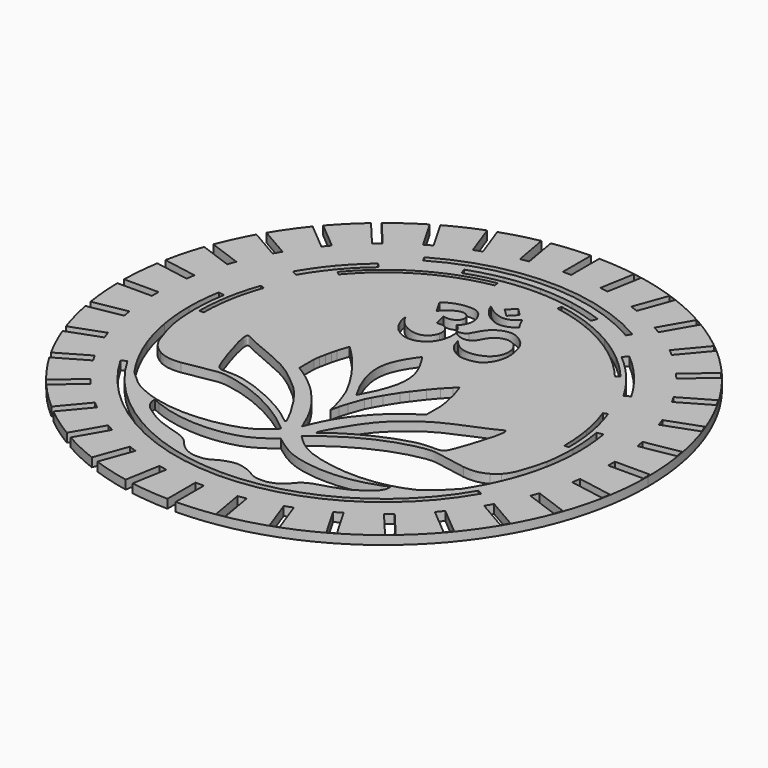
from build123d import *

# Parameters (mm, degrees)
F0_W     = 20
F0_H     = 4.75
F1_DEPTH = 5
F4_DEPTH = 12.5
F5_DEPTH = 12.5


with BuildPart() as f1:
    # F0 (on Top) → F1 (new body)
    with BuildSketch(Plane.XY):
        with BuildLine():
            ThreePointArc((1.597222, -149.991496), (106.629225, -105.499803), (150, 0))
            ThreePointArc((150, 0), (106.902409, 105.222978), (2.375, 149.981197))
            Line((2.375, 149.981197), (2.375, 130))
            Line((2.375, 130), (0, 130))
            Line((0, 130), (-2.375, 130))
            Line((-2.375, 130), (-2.375, 149.981197))
            ThreePointArc((-2.375, 149.981197), (-13.070418, 149.429462), (-23.699208, 148.115993))
            Line((-23.699208, 148.115993), (-20.241253, 128.504952))
            Line((-20.241253, 128.504952), (-24.91909, 127.680123))
            Line((-24.91909, 127.680123), (-28.377078, 147.291349))
            ThreePointArc((-28.377078, 147.291349), (-38.808675, 144.892673), (-49.042654, 141.756192))
            Line((-49.042654, 141.756192), (-42.254302, 123.105346))
            Line((-42.254302, 123.105346), (-46.717841, 121.480751))
            Line((-46.717841, 121.480751), (-53.506448, 140.132295))
            ThreePointArc((-53.506448, 140.132295), (-63.358495, 135.962131), (-72.88825, 131.100355))
            Line((-72.88825, 131.100355), (-62.995291, 113.965247))
            Line((-62.995291, 113.965247), (-67.108912, 111.590247))
            Line((-67.108912, 111.590247), (-77.002696, 128.726784))
            ThreePointArc((-77.002696, 128.726784), (-85.977844, 122.913833), (-94.516059, 116.476241))
            Line((-94.516059, 116.476241), (-81.834016, 101.362371))
            Line((-81.834016, 101.362371), (-85.472728, 98.30913))
            Line((-85.472728, 98.30913), (-98.156622, 113.425207))
            ThreePointArc((-98.156622, 113.425207), (-105.984694, 106.147278), (-113.274614, 98.330371))
            Line((-113.274614, 98.330371), (-98.198073, 85.679651))
            Line((-98.198073, 85.679651), (-101.251314, 82.04094))
            Line((-101.251314, 82.04094), (-116.331225, 94.694488))
            ThreePointArc((-116.331225, 94.694488), (-122.777115, 86.172966), (-128.600028, 77.2142))
            Line((-128.600028, 77.2142), (-111.590247, 67.393598))
            Line((-111.590247, 67.393598), (-113.965247, 63.279977))
            Line((-113.965247, 63.279977), (-130.980362, 73.103658))
            ThreePointArc((-130.980362, 73.103658), (-135.850845, 63.596761), (-140.032397, 53.767349))
            Line((-140.032397, 53.767349), (-121.603624, 47.059825))
            Line((-121.603624, 47.059825), (-123.22822, 42.596285))
            Line((-123.22822, 42.596285), (-141.664608, 49.306581))
            ThreePointArc((-141.664608, 49.306581), (-144.813896, 39.101606), (-147.229077, 28.698413))
            Line((-147.229077, 28.698413), (-127.933953, 25.296162))
            Line((-127.933953, 25.296162), (-128.758781, 20.618325))
            Line((-128.758781, 20.618325), (-148.063929, 24.022344))
            ThreePointArc((-148.063929, 24.022344), (-149.397831, 13.427143), (-149.974534, 2.763889))
            Line((-149.974534, 2.763889), (-130.388889, 2.763889))
            Line((-130.388889, 2.763889), (-130.388889, -1.986111))
            Line((-130.388889, -1.986111), (-149.986851, -1.986111))
            ThreePointArc((-149.986851, -1.986111), (-149.465453, -12.65221), (-148.186514, -23.254183))
            Line((-148.186514, -23.254183), (-128.893841, -19.852364))
            Line((-128.893841, -19.852364), (-128.069012, -24.530201))
            Line((-128.069012, -24.530201), (-147.375921, -27.93453))
            ThreePointArc((-147.375921, -27.93453), (-145.014723, -38.350099), (-141.918401, -48.571261))
            Line((-141.918401, -48.571261), (-123.494235, -41.865413))
            Line((-123.494235, -41.865413), (-121.86964, -46.328953))
            Line((-121.86964, -46.328953), (-140.309338, -53.040454))
            ThreePointArc((-140.309338, -53.040454), (-136.17882, -62.891405), (-131.357711, -72.423421))
            Line((-131.357711, -72.423421), (-114.354136, -62.606402))
            Line((-114.354136, -62.606402), (-111.979136, -66.720023))
            Line((-111.979136, -66.720023), (-128.99871, -76.546279))
            ThreePointArc((-128.99871, -76.546279), (-123.222343, -85.535105), (-116.820743, -94.089925))
            Line((-116.820743, -94.089925), (-101.75126, -81.445128))
            Line((-101.75126, -81.445128), (-98.698019, -85.083839))
            Line((-98.698019, -85.083839), (-113.783001, -97.741642))
            ThreePointArc((-113.783001, -97.741642), (-106.533732, -105.596231), (-98.743524, -112.914642))
            Line((-98.743524, -112.914642), (-86.06854, -97.809184))
            Line((-86.06854, -97.809184), (-82.429829, -100.862425))
            Line((-82.429829, -100.862425), (-95.118795, -115.984546))
            ThreePointArc((-95.118795, -115.984546), (-86.6141, -122.466313), (-77.669239, -128.325716))
            Line((-77.669239, -128.325716), (-67.782487, -111.201358))
            Line((-67.782487, -111.201358), (-63.668866, -113.576358))
            Line((-63.668866, -113.576358), (-73.56711, -130.720619))
            ThreePointArc((-73.56711, -130.720619), (-64.062721, -135.631736), (-54.23246, -139.852924))
            Line((-54.23246, -139.852924), (-47.448714, -121.214735))
            Line((-47.448714, -121.214735), (-42.985174, -122.839331))
            Line((-42.985174, -122.839331), (-49.777091, -141.499969))
            ThreePointArc((-49.777091, -141.499969), (-39.559543, -144.689469), (-29.140556, -147.142203))
            Line((-29.140556, -147.142203), (-25.685051, -127.545064))
            Line((-25.685051, -127.545064), (-21.007214, -128.369892))
            Line((-21.007214, -128.369892), (-24.466964, -147.991107))
            ThreePointArc((-24.466964, -147.991107), (-13.845159, -149.359672), (-3.152778, -149.966863))
            Line((-3.152778, -149.966863), (-3.152778, -130))
            Line((-3.152778, -130), (1.597222, -130))
            Line((1.597222, -130), (1.597222, -149.991496))
        make_face()
        Polygon((24.141312, -127.680123), (27.614275, -147.376278), (22.936439, -148.201107), (19.463475, -128.504952), align=None, mode=Mode.SUBTRACT)
        Polygon((45.940064, -121.480751), (52.780467, -140.274603), (48.316927, -141.899199), (41.476524, -123.105346), align=None, mode=Mode.SUBTRACT)
        Polygon((66.331134, -111.590247), (76.331134, -128.910755), (72.217513, -131.285755), (62.217513, -113.965247), align=None, mode=Mode.SUBTRACT)
        Polygon((84.69495, -98.30913), (97.550702, -113.630019), (93.911991, -116.68326), (81.056239, -101.362371), align=None, mode=Mode.SUBTRACT)
        Polygon((100.473536, -82.04094), (115.794425, -94.896692), (112.741184, -98.535403), (97.420295, -85.679651), align=None, mode=Mode.SUBTRACT)
        Polygon((113.187469, -63.279977), (130.507977, -73.279977), (128.132977, -77.393598), (110.812469, -67.393598), align=None, mode=Mode.SUBTRACT)
        Polygon((122.450442, -42.596285), (141.244294, -49.436688), (139.619699, -53.900227), (120.825846, -47.059825), align=None, mode=Mode.SUBTRACT)
        Polygon((127.981004, -20.618325), (147.677159, -24.091289), (146.85233, -28.769126), (127.156175, -25.296162), align=None, mode=Mode.SUBTRACT)
        with Locations((139.611111, -0.388889)):
            Rectangle(F0_W, F0_H, mode=Mode.SUBTRACT)
        Polygon((127.291234, 24.530201), (146.987389, 28.003164), (147.812218, 23.325327), (128.116063, 19.852364), align=None, mode=Mode.SUBTRACT)
        Polygon((121.091862, 46.328953), (139.885714, 53.169355), (141.51031, 48.705816), (122.716457, 41.865413), align=None, mode=Mode.SUBTRACT)
        Polygon((111.201358, 66.720023), (128.521866, 76.720023), (130.896866, 72.606402), (113.576358, 62.606402), align=None, mode=Mode.SUBTRACT)
        Polygon((20.229437, 128.369892), (23.7024, 148.066048), (28.380237, 147.241219), (24.907273, 127.545064), align=None, mode=Mode.SUBTRACT)
        Polygon((62.891088, 113.576358), (72.891088, 130.896866), (77.004709, 128.521866), (67.004709, 111.201358), align=None, mode=Mode.SUBTRACT)
        Polygon((42.207396, 122.839331), (49.047799, 141.633183), (53.511339, 140.008587), (46.670936, 121.214735), align=None, mode=Mode.SUBTRACT)
        Polygon((97.920241, 85.083839), (113.24113, 97.939591), (116.294371, 94.30088), (100.973482, 81.445128), align=None, mode=Mode.SUBTRACT)
        Polygon((81.652051, 100.862425), (94.507803, 116.183314), (98.146514, 113.130073), (85.290762, 97.809184), align=None, mode=Mode.SUBTRACT)
    extrude(amount=F1_DEPTH)

    # F3 (on face) → F4 (cut, symmetric)
    with BuildSketch(Plane(origin=(0, 0, 0), x_dir=(1, 0, 0), z_dir=(0, 0, -1))):
        with BuildLine():
            ThreePointArc((-57.608503, 99.780855), (-29.820356, 111.291082), (0, 115.217007))
            Line((0, 115.217007), (0, 118.357057))
            ThreePointArc((0, 118.357057), (-30.63306, 114.324138), (-59.178528, 102.500218))
            Line((-59.178528, 102.500218), (-57.608503, 99.780855))
        make_face()
        with BuildLine():
            ThreePointArc((0, 115.217007), (29.820356, 111.291082), (57.608503, 99.780855))
            Line((57.608503, 99.780855), (59.178528, 102.500218))
            ThreePointArc((59.178528, 102.500218), (30.63306, 114.324138), (0, 118.357057))
            Line((0, 118.357057), (0, 115.217007))
        make_face()
        with BuildLine():
            ThreePointArc((-99.780855, 57.608503), (-81.470727, 81.470727), (-57.608503, 99.780855))
            Line((-57.608503, 99.780855), (-59.178528, 102.500218))
            ThreePointArc((-59.178528, 102.500218), (-83.691077, 83.691077), (-102.500218, 59.178528))
            Line((-102.500218, 59.178528), (-99.780855, 57.608503))
        make_face()
        with BuildLine():
            ThreePointArc((57.608503, 99.780855), (81.470727, 81.470727), (99.780855, 57.608503))
            Line((99.780855, 57.608503), (102.500218, 59.178528))
            ThreePointArc((102.500218, 59.178528), (83.691077, 83.691077), (59.178528, 102.500218))
            Line((59.178528, 102.500218), (57.608503, 99.780855))
        make_face()
        with BuildLine():
            Line((59.178528, -102.500218), (57.608503, -99.780855))
            ThreePointArc((57.608503, -99.780855), (0, -115.217007), (-57.608503, -99.780855))
            Line((-57.608503, -99.780855), (-59.178528, -102.500218))
            ThreePointArc((-59.178528, -102.500218), (0, -118.357057), (59.178528, -102.500218))
        make_face()
    extrude(amount=F4_DEPTH, both=True, mode=Mode.SUBTRACT)

    # F2 (on Top) → F5 (cut, symmetric)
    with BuildSketch(Plane.XY):
        with BuildLine():
            add(Edge.make_bspline(
                [(-26.703293, 72.772757), (-22.478819, 76.516569), (-13.505565, 78.302662), (-8.586049, 77.175751), (-6.499787, 75.175449)],
                knots=[0, 0, 0, 0, 0.581389, 1, 1, 1, 1], degree=3))
            add(Edge.make_bspline(
                [(-26.703293, 72.772757), (-25.355081, 70.373524), (-24.053074, 68.074924), (-22.704862, 65.675691)],
                knots=[0, 0, 0, 0, 8.145907, 8.145907, 8.145907, 8.145907], degree=3))
            add(Edge.make_bspline(
                [(-8.665677, 69.281735), (-9.783125, 71.251235), (-13.605188, 73.021978), (-19.772128, 68.764412), (-21.8962, 66.595492), (-22.704862, 65.675691)],
                knots=[0, 0, 0, 0, 0.332513, 0.707051, 1, 1, 1, 1], degree=3))
            add(Edge.make_bspline(
                [(-17.057454, 63.531227), (-16.037357, 63.26761), (-13.208657, 62.663421), (-8.578156, 65.063049), (-8.277197, 67.8832), (-8.665677, 69.281735)],
                knots=[0, 0, 0, 0, 0.320478, 0.676624, 1, 1, 1, 1], degree=3))
            add(Edge.make_bspline(
                [(-15.444824, 56.62287), (-15.982367, 58.925656), (-16.519911, 61.228442), (-17.057454, 63.531227)],
                knots=[0, 0, 0, 0, 7.09408, 7.09408, 7.09408, 7.09408], degree=3))
            add(Edge.make_bspline(
                [(-7.991881, 49.536288), (-7.594286, 52.1168), (-9.312323, 56.461701), (-12.466869, 56.971069), (-15.444824, 56.62287)],
                knots=[0, 0, 0, 0, 0.508663, 1, 1, 1, 1], degree=3))
            add(Edge.make_bspline(
                [(-29.753646, 52.613709), (-28.553318, 49.875669), (-25.266547, 45.549492), (-15.312613, 41.506839), (-9.279541, 45.082696), (-7.991881, 49.536288)],
                knots=[0, 0, 0, 0, 0.315633, 0.654187, 1, 1, 1, 1], degree=3))
            add(Edge.make_bspline(
                [(-24.630969, 41.01808), (-26.457644, 42.921507), (-29.062424, 47.330559), (-29.671244, 50.90585), (-29.753646, 52.613709)],
                knots=[0, 0, 0, 0, 0.547939, 1, 1, 1, 1], degree=3))
            add(Edge.make_bspline(
                [(-2.568085, 54.219991), (-2.478607, 52.847017), (-2.376396, 49.888119), (-3.428155, 45.220364), (-6.026805, 41.186891), (-8.67628, 38.939767), (-12.542173, 37.245592), (-16.577244, 36.933956), (-20.991081, 38.095522), (-23.327493, 39.967105), (-24.630969, 41.01808)],
                knots=[0, 0, 0, 0, 0.124945, 0.257135, 0.38776, 0.499819, 0.62179, 0.742926, 0.869214, 1, 1, 1, 1], degree=3))
            add(Edge.make_bspline(
                [(19.814819, 63.531227), (18.768377, 63.637798), (16.005393, 63.028155), (12.611332, 61.256179), (10.143988, 57.191455), (9.248884, 55.056364), (7.358842, 52.780087), (3.834369, 51.865212), (0.587411, 52.562146), (-1.582146, 53.720386), (-2.568085, 54.219991)],
                knots=[0, 0, 0, 0, 0.129745, 0.263756, 0.408093, 0.51199, 0.624075, 0.750013, 0.873115, 1, 1, 1, 1], degree=3))
            add(Edge.make_bspline(
                [(2.779092, 49.023379), (3.524531, 48.139071), (5.061174, 46.316162), (8.41181, 44.063753), (12.929503, 42.815322), (18.32591, 43.76921), (22.435249, 45.5927), (25.43589, 48.537302), (27.143227, 52.461491), (27.136221, 57.967533), (24.075212, 62.45953), (21.486653, 63.253537), (19.814819, 63.531227)],
                knots=[0, 0, 0, 0, 0.088628, 0.182697, 0.284338, 0.39447, 0.494693, 0.589628, 0.686383, 0.795998, 0.901602, 1, 1, 1, 1], degree=3))
            add(Edge.make_bspline(
                [(29.083719, 56.863476), (29.346624, 55.498138), (29.946058, 51.835685), (28.788033, 45.586509), (26.804438, 42.261139), (24.342062, 39.384339), (20.845119, 37.95796), (15.851711, 37.257572), (10.876852, 37.898382), (5.88339, 41.831034), (3.659308, 45.212339), (3.069999, 47.763849), (2.779092, 49.023379)],
                knots=[0, 0, 0, 0, 0.104459, 0.221836, 0.313636, 0.401904, 0.491563, 0.595441, 0.699744, 0.815334, 0.908841, 1, 1, 1, 1], degree=3))
            add(Edge.make_bspline(
                [(2.009738, 57.852648), (3.693849, 60.468544), (5.726443, 66.167234), (15.863503, 71.372649), (23.67625, 67.30442), (27.644872, 62.48758), (28.609513, 58.71806), (29.083719, 56.863476)],
                knots=[0, 0, 0, 0, 0.217271, 0.445619, 0.650372, 0.828044, 1, 1, 1, 1], degree=3))
            add(Edge.make_bspline(
                [(-3.712958, 56.326561), (-3.045915, 55.933479), (-1.286406, 55.653666), (1.058829, 56.729218), (2.009738, 57.852648)],
                knots=[0, 0, 0, 0, 0.436713, 1, 1, 1, 1], degree=3))
            add(Edge.make_bspline(
                [(-7.261419, 60.502313), (-6.41553, 60.155282), (-4.686406, 58.60729), (-4.184914, 57.1977), (-3.712958, 56.326561)],
                knots=[0, 0, 0, 0, 0.519128, 1, 1, 1, 1], degree=3))
            add(Edge.make_bspline(
                [(-6.499787, 75.175449), (-4.902218, 72.844208), (-2.580657, 68.502349), (-4.714982, 62.642939), (-7.261419, 60.502313)],
                knots=[0, 0, 0, 0, 0.481783, 1, 1, 1, 1], degree=3))
        make_face()
        with BuildLine():
            add(Edge.make_bspline(
                [(-6.618558, 84.143944), (-3.438113, 81.399173), (3.917643, 77.195458), (9.457943, 79.525754), (12.442335, 82.793348)],
                knots=[0, 0, 0, 0, 0.52571, 1, 1, 1, 1], degree=3))
            add(Edge.make_bspline(
                [(15.862403, 76.34531), (13.959511, 74.267434), (7.616297, 70.926623), (-2.460375, 76.240025), (-5.876792, 82.00591), (-6.618558, 84.143944)],
                knots=[0, 0, 0, 0, 0.325363, 0.68111, 1, 1, 1, 1], degree=3))
            add(Edge.make_bspline(
                [(12.442335, 82.793348), (13.444393, 80.418892), (14.272179, 78.545474), (15.862403, 76.34531)],
                knots=[0, 0, 0, 0, 7.298908, 7.298908, 7.298908, 7.298908], degree=3))
        make_face()
        Polygon((8.61929, 85.590638), (4.404083, 89.894883), (0.156227, 85.538112), (4.46861, 81.333535), align=None)
        with BuildLine():
            Line((18.667179, 105.866833), (19.274948, 109.313661))
            ThreePointArc((19.274948, 109.313661), (9.674287, 110.577611), (0, 111))
            Line((0, 111), (0, 107.5))
            ThreePointArc((0, 107.5), (9.369242, 107.09093), (18.667179, 105.866833))
        make_face()
        with BuildLine():
            Line((0, 107.5), (0, 111))
            ThreePointArc((0, 111), (-9.674287, 110.577611), (-19.274948, 109.313661))
            Line((-19.274948, 109.313661), (-18.667179, 105.866833))
            ThreePointArc((-18.667179, 105.866833), (-9.369242, 107.09093), (0, 107.5))
        make_face()
        with BuildLine():
            Line((-18.667179, 105.866833), (-19.274948, 109.313661))
            ThreePointArc((-19.274948, 109.313661), (-28.728914, 107.217767), (-37.964236, 104.305881))
            Line((-37.964236, 104.305881), (-36.767165, 101.016957))
            ThreePointArc((-36.767165, 101.016957), (-27.823047, 103.837026), (-18.667179, 105.866833))
        make_face()
        with BuildLine():
            Line((36.767165, 101.016957), (37.964236, 104.305881))
            ThreePointArc((37.964236, 104.305881), (28.728914, 107.217767), (19.274948, 109.313661))
            Line((19.274948, 109.313661), (18.667179, 105.866833))
            ThreePointArc((18.667179, 105.866833), (27.823047, 103.837026), (36.767165, 101.016957))
        make_face()
        with BuildLine():
            ThreePointArc((88.767604, -51.25), (91.318275, -46.553438), (93.620677, -41.730311))
            add(Edge.make_bspline(
                [(93.620677, -41.730311), (90.555624, -43.531707), (86.44454, -44.750247), (80.26686, -43.949023)],
                knots=[0.65431, 0.65431, 0.65431, 0.65431, 1, 1, 1, 1], degree=3))
            add(Edge.make_bspline(
                [(80.26686, -43.949023), (63.634888, -41.093014), (61.069282, -38.499597), (26.838655, -47.513978), (5.753011, -65.722443)],
                knots=[0, 0, 0, 0, 0.392786, 1, 1, 1, 1], degree=3))
            add(Edge.make_bspline(
                [(5.753011, -65.722443), (12.107129, -72.466477), (23.636298, -79.03376), (51.209658, -82.137114), (66.01574, -78.41028)],
                knots=[0, 0, 0, 0, 0.403723, 0.874059, 0.874059, 0.874059, 0.874059], degree=3))
            ThreePointArc((66.01574, -78.41028), (72.538466, -72.418375), (78.519555, -65.88573))
            ThreePointArc((78.519555, -65.88573), (83.963085, -58.791585), (88.767604, -51.25))
        make_face()
        with BuildLine():
            ThreePointArc((-78.519555, -65.88573), (-72.538466, -72.418375), (-66.01574, -78.41028))
            add(Edge.make_bspline(
                [(-5.753011, -65.722443), (-12.107129, -72.466477), (-23.636298, -79.03376), (-51.209658, -82.137114), (-66.01574, -78.41028)],
                knots=[0, 0, 0, 0, 0.403723, 0.874059, 0.874059, 0.874059, 0.874059], degree=3))
            add(Edge.make_bspline(
                [(-80.26686, -43.949023), (-63.634888, -41.093014), (-61.069282, -38.499597), (-26.838655, -47.513978), (-5.753011, -65.722443)],
                knots=[0, 0, 0, 0, 0.392786, 1, 1, 1, 1], degree=3))
            add(Edge.make_bspline(
                [(-93.620677, -41.730311), (-90.555624, -43.531707), (-86.44454, -44.750247), (-80.26686, -43.949023)],
                knots=[0.65431, 0.65431, 0.65431, 0.65431, 1, 1, 1, 1], degree=3))
            ThreePointArc((-93.620677, -41.730311), (-91.318275, -46.553438), (-88.767604, -51.25))
            ThreePointArc((-88.767604, -51.25), (-83.963085, -58.791585), (-78.519555, -65.88573))
        make_face()
        with BuildLine():
            add(Edge.make_bspline(
                [(-8.756669, -58.829643), (-8.512867, -57.277238), (-20.68578, -35.778175), (-31.846786, -26.836212), (-44.0248, -16.558039), (-68.270317, -8.056344), (-76.638483, -2.04947), (-66.875449, -32.037339), (-63.386402, -39.253539), (-50.289925, -36.005567), (-17.179196, -51.155717), (-8.903584, -59.765119), (-8.756669, -58.829643)],
                knots=[0, 0, 0, 0, 0.119539, 0.219887, 0.318313, 0.445689, 0.496312, 0.623336, 0.691915, 0.774065, 0.927966, 1, 1, 1, 1], degree=3))
        make_face()
        Polygon((-31.268656, 14.674164), (-31.431369, 14.299355), (-33.409711, 8.364327), (-34.142431, 5.433451), (-34.875151, 1.989669), (-35.607871, -1.454111), (-36.051683, -4.752926), (-36.051683, -8.11421), (-36.051683, -15.138219), (-33.340007, -16.868144), (-30.320914, -18.870603), (-27.486667, -21.027096), (-24.559997, -23.368433), (-21.078799, -26.418332), (-18.275356, -29.190967), (-15.225458, -32.641355), (-13.253807, -34.982692), (-10.727628, -38.094204), (-8.571135, -41.298136), (-6.507062, -44.563685), (-3.906751, -49.339846), (-0.203492, -57.748422), (0, -58.401939), (0, -38.022086), (-1.109756, -33.216286), (-2.403652, -28.718457), (-5.299515, -20.647008), (-6.951439, -17.476365), (-9.515956, -12.786962), (-13.785807, -6.031676), (-16.401676, -2.424505), (-21.078799, 3.663297), (-25.235467, 8.559444), (-29.199015, 12.65252), (-30.831063, 14.299355), align=None)
        Polygon((1.109756, -33.216286), (0, -38.022086), (0, -58.401939), (0.203492, -57.748422), (3.906751, -49.339846), (6.507062, -44.563685), (8.571135, -41.298136), (10.727628, -38.094204), (13.253807, -34.982692), (15.225458, -32.641355), (18.275356, -29.190967), (21.078799, -26.418332), (24.559997, -23.368433), (27.486667, -21.027096), (30.320914, -18.870603), (33.340007, -16.868144), (36.051683, -15.138219), (36.051683, -8.11421), (36.051683, -4.752926), (35.607871, -1.454111), (34.875151, 1.989669), (34.142431, 5.433451), (33.409711, 8.364327), (31.431369, 14.299355), (31.268656, 14.674164), (30.831063, 14.299355), (29.199015, 12.65252), (25.235467, 8.559444), (21.078799, 3.663297), (16.401676, -2.424505), (13.785807, -6.031676), (9.515956, -12.786962), (6.951439, -17.476365), (5.299515, -20.647008), (2.403652, -28.718457), align=None)
        with BuildLine():
            add(Edge.make_bspline(
                [(0, 27.158394), (5.556337, 18.972242), (11.233916, 6.603466), (5.867204, -9.316608), (0, -19.678826)],
                knots=[0, 0, 0, 0, 0.474526, 1, 1, 1, 1], degree=3))
            add(Edge.make_bspline(
                [(0, 27.158394), (-4.03931, 21.755195), (-13.577049, 7.236363), (-4.287768, -12.839762), (0, -19.678826)],
                knots=[0, 0, 0, 0, 0.470917, 1, 1, 1, 1], degree=3))
        make_face()
        with BuildLine():
            add(Edge.make_bspline(
                [(8.756669, -58.829643), (8.512867, -57.277238), (20.68578, -35.778175), (31.846786, -26.836212), (44.0248, -16.558039), (68.270317, -8.056344), (76.638483, -2.04947), (66.875449, -32.037339), (63.386402, -39.253539), (50.289925, -36.005567), (17.179196, -51.155717), (8.903584, -59.765119), (8.756669, -58.829643)],
                knots=[0, 0, 0, 0, 0.119539, 0.219887, 0.318313, 0.445689, 0.496312, 0.623336, 0.691915, 0.774065, 0.927966, 1, 1, 1, 1], degree=3))
        make_face()
        with BuildLine():
            ThreePointArc((51.25, -88.767604), (57.437831, -84.894909), (63.334342, -80.591632))
            add(Edge.make_bspline(
                [(0, -73.347926), (8.360746, -79.816064), (20.263876, -86.223745), (48.140199, -86.722674), (63.334342, -80.591632)],
                knots=[0, 0, 0, 0, 0.424708, 0.957273, 0.957273, 0.957273, 0.957273], degree=3))
            add(Edge.make_bspline(
                [(0, -73.347926), (-8.360746, -79.816064), (-20.263876, -86.223745), (-48.140199, -86.722674), (-63.334342, -80.591632)],
                knots=[0, 0, 0, 0, 0.424708, 0.957273, 0.957273, 0.957273, 0.957273], degree=3))
            ThreePointArc((-63.334342, -80.591632), (-57.437831, -84.894909), (-51.25, -88.767604))
            ThreePointArc((-51.25, -88.767604), (-43.318372, -92.896548), (-35.057065, -96.318494))
            ThreePointArc((-35.057065, -96.318494), (-26.528952, -99.007397), (-17.798938, -100.942795))
            ThreePointArc((-17.798938, -100.942795), (-8.933464, -102.109957), (0, -102.5))
            ThreePointArc((0, -102.5), (8.933464, -102.109957), (17.798938, -100.942795))
            ThreePointArc((17.798938, -100.942795), (26.528952, -99.007397), (35.057065, -96.318494))
            ThreePointArc((35.057065, -96.318494), (43.318372, -92.896548), (51.25, -88.767604))
        make_face()
        with BuildLine():
            Line((-104.305881, -37.964236), (-101.016957, -36.767165))
            ThreePointArc((-101.016957, -36.767165), (-103.837026, -27.823047), (-105.866833, -18.667179))
            Line((-105.866833, -18.667179), (-109.313661, -19.274948))
            ThreePointArc((-109.313661, -19.274948), (-107.217767, -28.728914), (-104.305881, -37.964236))
        make_face()
        with BuildLine():
            add(Edge.make_bspline(
                [(-71.711666, -76.697047), (-73.761937, -75.97472), (-75.799944, -75.136756), (-77.813051, -74.171283)],
                knots=[0.934493, 0.934493, 0.934493, 0.934493, 1, 1, 1, 1], degree=3))
            ThreePointArc((-71.711666, -76.697047), (-76.212247, -72.226681), (-80.434667, -67.492699))
            ThreePointArc((-80.434667, -67.492699), (-86.010965, -60.225526), (-90.932667, -52.5))
            ThreePointArc((-90.932667, -52.5), (-94.530293, -45.705839), (-97.621154, -38.666655))
            add(Edge.make_bspline(
                [(-106.178021, -16.807077), (-102.808414, -30.867097), (-100.746034, -35.563512), (-97.621154, -38.666655)],
                knots=[0, 0, 0, 0, 0.478354, 0.478354, 0.478354, 0.478354], degree=3))
            ThreePointArc((-106.178021, -16.807077), (-106.026506, -17.73781), (-105.866833, -18.667179))
            ThreePointArc((-105.866833, -18.667179), (-103.837026, -27.823047), (-101.016957, -36.767165))
            ThreePointArc((-101.016957, -36.767165), (-97.428087, -45.431463), (-93.097731, -53.75))
            ThreePointArc((-93.097731, -53.75), (-88.058845, -61.659467), (-82.349778, -69.099668))
            ThreePointArc((-82.349778, -69.099668), (-80.121553, -71.671381), (-77.813051, -74.171283))
        make_face()
        with BuildLine():
            Line((-80.434667, -67.492699), (-78.519555, -65.88573))
            ThreePointArc((-78.519555, -65.88573), (-83.963085, -58.791585), (-88.767604, -51.25))
            Line((-88.767604, -51.25), (-90.932667, -52.5))
            ThreePointArc((-90.932667, -52.5), (-86.010965, -60.225526), (-80.434667, -67.492699))
        make_face()
        with BuildLine():
            Line((-90.932667, -52.5), (-88.767604, -51.25))
            ThreePointArc((-88.767604, -51.25), (-91.318275, -46.553438), (-93.620677, -41.730311))
            add(Edge.make_bspline(
                [(-97.621154, -38.666655), (-97.114355, -39.169929), (-95.901522, -40.216333), (-94.492926, -41.217672), (-93.620677, -41.730311)],
                knots=[0.478354, 0.478354, 0.478354, 0.478354, 0.555934, 0.65431, 0.65431, 0.65431, 0.65431], degree=3))
            ThreePointArc((-97.621154, -38.666655), (-94.530293, -45.705839), (-90.932667, -52.5))
        make_face()
        with BuildLine():
            Line((-96.12882, -55.5), (-93.097731, -53.75))
            ThreePointArc((-93.097731, -53.75), (-97.428087, -45.431463), (-101.016957, -36.767165))
            Line((-101.016957, -36.767165), (-104.305881, -37.964236))
            ThreePointArc((-104.305881, -37.964236), (-100.600164, -46.910627), (-96.12882, -55.5))
        make_face()
        with BuildLine():
            Line((-83.813158, -70.32759), (-82.349778, -69.099668))
            ThreePointArc((-82.349778, -69.099668), (-88.058845, -61.659467), (-93.097731, -53.75))
            Line((-93.097731, -53.75), (-96.12882, -55.5))
            ThreePointArc((-96.12882, -55.5), (-93.450958, -59.899236), (-90.571918, -64.169523))
            add(Edge.make_bspline(
                [(-83.813158, -70.32759), (-85.615706, -68.876625), (-87.76621, -66.927467), (-90.571918, -64.169523)],
                knots=[9.205673, 9.205673, 9.205673, 9.205673, 16.211844, 16.211844, 16.211844, 16.211844], degree=3))
        make_face()
        with BuildLine():
            add(Edge.make_bspline(
                [(-77.813051, -74.171283), (-79.677009, -73.280447), (-81.444722, -72.234067), (-83.813158, -70.32759)],
                knots=[0, 0, 0, 0, 9.205673, 9.205673, 9.205673, 9.205673], degree=3))
            ThreePointArc((-77.813051, -74.171283), (-80.121553, -71.671381), (-82.349778, -69.099668))
            Line((-82.349778, -69.099668), (-83.813158, -70.32759))
        make_face()
        with BuildLine():
            add(Edge.make_bspline(
                [(-66.01574, -78.41028), (-67.918206, -77.931411), (-69.820155, -77.36344), (-71.711666, -76.697047)],
                knots=[0.874059, 0.874059, 0.874059, 0.874059, 0.934493, 0.934493, 0.934493, 0.934493], degree=3))
            ThreePointArc((-66.01574, -78.41028), (-72.538466, -72.418375), (-78.519555, -65.88573))
            Line((-78.519555, -65.88573), (-80.434667, -67.492699))
            ThreePointArc((-80.434667, -67.492699), (-76.212247, -72.226681), (-71.711666, -76.697047))
        make_face()
        with BuildLine():
            ThreePointArc((-51.25, -88.767604), (-57.437831, -84.894909), (-63.334342, -80.591632))
            add(Edge.make_bspline(
                [(-63.334342, -80.591632), (-64.38469, -80.167802), (-65.433535, -79.713348), (-66.479141, -79.226755)],
                knots=[0.957273, 0.957273, 0.957273, 0.957273, 0.994088, 0.994088, 0.994088, 0.994088], degree=3))
            Line((-66.479141, -79.226755), (-67.087328, -79.951564))
            add(Edge.make_bspline(
                [(-67.087328, -79.951564), (-67.094447, -80.23865), (-67.080133, -80.524066), (-67.045747, -80.807597)],
                knots=[0.030613, 0.030613, 0.030613, 0.030613, 0.058197, 0.058197, 0.058197, 0.058197], degree=3))
            ThreePointArc((-67.045747, -80.807597), (-59.986879, -86.177574), (-52.5, -90.932667))
            Line((-52.5, -90.932667), (-51.25, -88.767604))
        make_face()
        with BuildLine():
            Line((-67.087328, -79.951564), (-66.479141, -79.226755))
            add(Edge.make_bspline(
                [(-66.479141, -79.226755), (-66.647036, -79.148622), (-66.814847, -79.06966), (-66.982567, -78.989863)],
                knots=[0.994088, 0.994088, 0.994088, 0.994088, 1, 1, 1, 1], degree=3))
            add(Edge.make_bspline(
                [(-66.982567, -78.989863), (-67.045127, -79.312286), (-67.079427, -79.632953), (-67.087328, -79.951564)],
                knots=[0, 0, 0, 0, 0.030613, 0.030613, 0.030613, 0.030613], degree=3))
        make_face()
        with BuildLine():
            ThreePointArc((-35.912115, -98.667725), (-44.374917, -95.162318), (-52.5, -90.932667))
            ThreePointArc((-52.5, -90.932667), (-59.986879, -86.177574), (-67.045747, -80.807597))
            add(Edge.make_bspline(
                [(-67.045747, -80.807597), (-66.789132, -82.923545), (-65.414647, -84.934435), (-63.488221, -86.749616)],
                knots=[0.058197, 0.058197, 0.058197, 0.058197, 0.26405, 0.26405, 0.26405, 0.26405], degree=3))
            ThreePointArc((-63.488221, -86.749616), (-59.358622, -89.625911), (-55.098933, -92.305783))
            add(Edge.make_bspline(
                [(-55.098933, -92.305783), (-49.307914, -95.18419), (-43.813774, -96.524823), (-38.259972, -98.26038)],
                knots=[0.51238, 0.51238, 0.51238, 0.51238, 1, 1, 1, 1], degree=3))
            add(Edge.make_bspline(
                [(-38.259972, -98.26038), (-34.076356, -99.945451), (-32.720586, -101.275105), (-31.434108, -102.801492)],
                knots=[0, 0, 0, 0, 0.393703, 0.393703, 0.393703, 0.393703], degree=3))
            ThreePointArc((-31.434108, -102.801492), (-25.097486, -104.52926), (-18.667179, -105.866833))
            ThreePointArc((-18.667179, -105.866833), (-14.023993, -106.581319), (-9.354025, -107.09226))
            add(Edge.make_bspline(
                [(-9.354025, -107.09226), (-7.975369, -106.316325), (-6.313653, -105.504483), (-3.980111, -104.924538)],
                knots=[0.6112, 0.6112, 0.6112, 0.6112, 0.871759, 0.871759, 0.871759, 0.871759], degree=3))
            ThreePointArc((-3.980111, -104.924538), (-11.132548, -104.408172), (-18.233059, -103.404814))
            ThreePointArc((-18.233059, -103.404814), (-27.176, -101.422212), (-35.912115, -98.667725))
        make_face()
        with BuildLine():
            ThreePointArc((-35.057065, -96.318494), (-43.318372, -92.896548), (-51.25, -88.767604))
            Line((-51.25, -88.767604), (-52.5, -90.932667))
            ThreePointArc((-52.5, -90.932667), (-44.374917, -95.162318), (-35.912115, -98.667725))
            Line((-35.912115, -98.667725), (-35.057065, -96.318494))
        make_face()
        with BuildLine():
            ThreePointArc((-17.798938, -100.942795), (-26.528952, -99.007397), (-35.057065, -96.318494))
            Line((-35.057065, -96.318494), (-35.912115, -98.667725))
            ThreePointArc((-35.912115, -98.667725), (-27.176, -101.422212), (-18.233059, -103.404814))
            Line((-18.233059, -103.404814), (-17.798938, -100.942795))
        make_face()
        with BuildLine():
            add(Edge.make_bspline(
                [(-20.674706, -109.764077), (-18.94088, -109.861758), (-17.573352, -109.862047), (-16.441869, -109.775521)],
                knots=[0, 0, 0, 0, 0.155797, 0.155797, 0.155797, 0.155797], degree=3))
            ThreePointArc((-16.441869, -109.775521), (-17.859901, -109.553749), (-19.274948, -109.313661))
            ThreePointArc((-19.274948, -109.313661), (-22.473618, -108.701134), (-25.652941, -107.995031))
            add(Edge.make_bspline(
                [(-25.652941, -107.995031), (-24.300318, -108.73328), (-22.671536, -109.359314), (-20.674706, -109.764077)],
                knots=[0.806024, 0.806024, 0.806024, 0.806024, 1, 1, 1, 1], degree=3))
        make_face()
        with BuildLine():
            ThreePointArc((-25.652941, -107.995031), (-22.473618, -108.701134), (-19.274948, -109.313661))
            Line((-19.274948, -109.313661), (-18.667179, -105.866833))
            ThreePointArc((-18.667179, -105.866833), (-25.097486, -104.52926), (-31.434108, -102.801492))
            add(Edge.make_bspline(
                [(-31.434108, -102.801492), (-31.174065, -103.11003), (-29.841418, -104.750248), (-27.973184, -106.728662), (-25.652941, -107.995031)],
                knots=[0.393703, 0.393703, 0.393703, 0.393703, 0.473284, 0.806024, 0.806024, 0.806024, 0.806024], degree=3))
        make_face()
        with BuildLine():
            ThreePointArc((-19.274948, -109.313661), (-17.859901, -109.553749), (-16.441869, -109.775521))
            add(Edge.make_bspline(
                [(-16.441869, -109.775521), (-14.17836, -109.602427), (-12.251238, -108.841852), (-10.114548, -107.520298), (-9.354025, -107.09226)],
                knots=[0.155797, 0.155797, 0.155797, 0.155797, 0.467465, 0.6112, 0.6112, 0.6112, 0.6112], degree=3))
            ThreePointArc((-9.354025, -107.09226), (-14.023993, -106.581319), (-18.667179, -105.866833))
            Line((-18.667179, -105.866833), (-19.274948, -109.313661))
        make_face()
        with BuildLine():
            Line((0, -104.268685), (0, -102.5))
            ThreePointArc((0, -102.5), (-8.933464, -102.109957), (-17.798938, -100.942795))
            Line((-17.798938, -100.942795), (-18.233059, -103.404814))
            ThreePointArc((-18.233059, -103.404814), (-11.132548, -104.408172), (-3.980111, -104.924538))
            add(Edge.make_bspline(
                [(-3.980111, -104.924538), (-2.831598, -104.639103), (-1.520344, -104.409843), (0, -104.268685)],
                knots=[0.871759, 0.871759, 0.871759, 0.871759, 1, 1, 1, 1], degree=3))
        make_face()
        with BuildLine():
            ThreePointArc((3.980111, -104.924538), (11.132548, -104.408172), (18.233059, -103.404814))
            Line((18.233059, -103.404814), (17.798938, -100.942795))
            ThreePointArc((17.798938, -100.942795), (8.933464, -102.109957), (0, -102.5))
            Line((0, -102.5), (0, -104.268685))
            add(Edge.make_bspline(
                [(3.980111, -104.924538), (2.831598, -104.639103), (1.520344, -104.409843), (0, -104.268685)],
                knots=[0.871759, 0.871759, 0.871759, 0.871759, 1, 1, 1, 1], degree=3))
        make_face()
        with BuildLine():
            ThreePointArc((16.441869, -109.775521), (17.859901, -109.553749), (19.274948, -109.313661))
            Line((19.274948, -109.313661), (18.667179, -105.866833))
            ThreePointArc((18.667179, -105.866833), (14.023993, -106.581319), (9.354025, -107.09226))
            add(Edge.make_bspline(
                [(16.441869, -109.775521), (14.17836, -109.602427), (12.251238, -108.841852), (10.114548, -107.520298), (9.354025, -107.09226)],
                knots=[0.155797, 0.155797, 0.155797, 0.155797, 0.467465, 0.6112, 0.6112, 0.6112, 0.6112], degree=3))
        make_face()
        with BuildLine():
            ThreePointArc((19.274948, -109.313661), (22.473618, -108.701134), (25.652941, -107.995031))
            add(Edge.make_bspline(
                [(31.434108, -102.801492), (31.174065, -103.11003), (29.841418, -104.750248), (27.973184, -106.728662), (25.652941, -107.995031)],
                knots=[0.393703, 0.393703, 0.393703, 0.393703, 0.473284, 0.806024, 0.806024, 0.806024, 0.806024], degree=3))
            ThreePointArc((31.434108, -102.801492), (25.097486, -104.52926), (18.667179, -105.866833))
            Line((18.667179, -105.866833), (19.274948, -109.313661))
        make_face()
        with BuildLine():
            ThreePointArc((55.098933, -92.305783), (59.358622, -89.625911), (63.488221, -86.749616))
            add(Edge.make_bspline(
                [(67.045747, -80.807597), (66.789132, -82.923545), (65.414647, -84.934435), (63.488221, -86.749616)],
                knots=[0.058197, 0.058197, 0.058197, 0.058197, 0.26405, 0.26405, 0.26405, 0.26405], degree=3))
            ThreePointArc((67.045747, -80.807597), (59.986879, -86.177574), (52.5, -90.932667))
            ThreePointArc((52.5, -90.932667), (44.374917, -95.162318), (35.912115, -98.667725))
            ThreePointArc((35.912115, -98.667725), (27.176, -101.422212), (18.233059, -103.404814))
            ThreePointArc((18.233059, -103.404814), (11.132548, -104.408172), (3.980111, -104.924538))
            add(Edge.make_bspline(
                [(9.354025, -107.09226), (7.975369, -106.316325), (6.313653, -105.504483), (3.980111, -104.924538)],
                knots=[0.6112, 0.6112, 0.6112, 0.6112, 0.871759, 0.871759, 0.871759, 0.871759], degree=3))
            ThreePointArc((9.354025, -107.09226), (14.023993, -106.581319), (18.667179, -105.866833))
            ThreePointArc((18.667179, -105.866833), (25.097486, -104.52926), (31.434108, -102.801492))
            add(Edge.make_bspline(
                [(38.259972, -98.26038), (34.076356, -99.945451), (32.720586, -101.275105), (31.434108, -102.801492)],
                knots=[0, 0, 0, 0, 0.393703, 0.393703, 0.393703, 0.393703], degree=3))
            add(Edge.make_bspline(
                [(55.098933, -92.305783), (49.307914, -95.18419), (43.813774, -96.524823), (38.259972, -98.26038)],
                knots=[0.51238, 0.51238, 0.51238, 0.51238, 1, 1, 1, 1], degree=3))
        make_face()
        with BuildLine():
            ThreePointArc((18.233059, -103.404814), (27.176, -101.422212), (35.912115, -98.667725))
            Line((35.912115, -98.667725), (35.057065, -96.318494))
            ThreePointArc((35.057065, -96.318494), (26.528952, -99.007397), (17.798938, -100.942795))
            Line((17.798938, -100.942795), (18.233059, -103.404814))
        make_face()
        with BuildLine():
            add(Edge.make_bspline(
                [(25.652941, -107.995031), (24.300318, -108.73328), (22.671536, -109.359314), (20.674706, -109.764077)],
                knots=[0.806024, 0.806024, 0.806024, 0.806024, 1, 1, 1, 1], degree=3))
            ThreePointArc((25.652941, -107.995031), (22.473618, -108.701134), (19.274948, -109.313661))
            ThreePointArc((19.274948, -109.313661), (17.859901, -109.553749), (16.441869, -109.775521))
            add(Edge.make_bspline(
                [(20.674706, -109.764077), (18.94088, -109.861758), (17.573352, -109.862047), (16.441869, -109.775521)],
                knots=[0, 0, 0, 0, 0.155797, 0.155797, 0.155797, 0.155797], degree=3))
        make_face()
        with BuildLine():
            ThreePointArc((35.912115, -98.667725), (44.374917, -95.162318), (52.5, -90.932667))
            Line((52.5, -90.932667), (51.25, -88.767604))
            ThreePointArc((51.25, -88.767604), (43.318372, -92.896548), (35.057065, -96.318494))
            Line((35.057065, -96.318494), (35.912115, -98.667725))
        make_face()
        with BuildLine():
            ThreePointArc((52.5, -90.932667), (59.986879, -86.177574), (67.045747, -80.807597))
            add(Edge.make_bspline(
                [(67.087328, -79.951564), (67.094447, -80.23865), (67.080133, -80.524066), (67.045747, -80.807597)],
                knots=[0.030613, 0.030613, 0.030613, 0.030613, 0.058197, 0.058197, 0.058197, 0.058197], degree=3))
            Line((67.087328, -79.951564), (66.479141, -79.226755))
            add(Edge.make_bspline(
                [(63.334342, -80.591632), (64.38469, -80.167802), (65.433535, -79.713348), (66.479141, -79.226755)],
                knots=[0.957273, 0.957273, 0.957273, 0.957273, 0.994088, 0.994088, 0.994088, 0.994088], degree=3))
            ThreePointArc((63.334342, -80.591632), (57.437831, -84.894909), (51.25, -88.767604))
            Line((51.25, -88.767604), (52.5, -90.932667))
        make_face()
        with BuildLine():
            Line((66.479141, -79.226755), (67.087328, -79.951564))
            add(Edge.make_bspline(
                [(66.982567, -78.989863), (67.045127, -79.312286), (67.079427, -79.632953), (67.087328, -79.951564)],
                knots=[0, 0, 0, 0, 0.030613, 0.030613, 0.030613, 0.030613], degree=3))
            add(Edge.make_bspline(
                [(66.479141, -79.226755), (66.647036, -79.148622), (66.814847, -79.06966), (66.982567, -78.989863)],
                knots=[0.994088, 0.994088, 0.994088, 0.994088, 1, 1, 1, 1], degree=3))
        make_face()
        with BuildLine():
            ThreePointArc((71.711666, -76.697047), (76.212247, -72.226681), (80.434667, -67.492699))
            Line((80.434667, -67.492699), (78.519555, -65.88573))
            ThreePointArc((78.519555, -65.88573), (72.538466, -72.418375), (66.01574, -78.41028))
            add(Edge.make_bspline(
                [(66.01574, -78.41028), (67.918206, -77.931411), (69.820155, -77.36344), (71.711666, -76.697047)],
                knots=[0.874059, 0.874059, 0.874059, 0.874059, 0.934493, 0.934493, 0.934493, 0.934493], degree=3))
        make_face()
        with BuildLine():
            add(Edge.make_bspline(
                [(77.813051, -74.171283), (79.540808, -73.131345), (81.368831, -71.831304), (83.478886, -70.047103)],
                knots=[0, 0, 0, 0, 8.984423, 8.984423, 8.984423, 8.984423], degree=3))
            Line((83.478886, -70.047103), (82.349778, -69.099668))
            ThreePointArc((82.349778, -69.099668), (80.121553, -71.671381), (77.813051, -74.171283))
        make_face()
        with BuildLine():
            ThreePointArc((92.720053, -61.024518), (94.464831, -58.287184), (96.12882, -55.5))
            Line((96.12882, -55.5), (93.097731, -53.75))
            ThreePointArc((93.097731, -53.75), (88.058845, -61.659467), (82.349778, -69.099668))
            Line((82.349778, -69.099668), (83.478886, -70.047103))
            add(Edge.make_bspline(
                [(83.478886, -70.047103), (86.036854, -67.884159), (89.0093, -65.009689), (92.720053, -61.024518)],
                knots=[8.984423, 8.984423, 8.984423, 8.984423, 19.876018, 19.876018, 19.876018, 19.876018], degree=3))
        make_face()
        with BuildLine():
            ThreePointArc((101.016957, -36.767165), (103.837026, -27.823047), (105.866833, -18.667179))
            ThreePointArc((105.866833, -18.667179), (106.026506, -17.73781), (106.178021, -16.807077))
            add(Edge.make_bspline(
                [(106.178021, -16.807077), (102.808414, -30.867097), (100.746034, -35.563512), (97.621154, -38.666655)],
                knots=[0, 0, 0, 0, 0.478354, 0.478354, 0.478354, 0.478354], degree=3))
            ThreePointArc((97.621154, -38.666655), (94.530293, -45.705839), (90.932667, -52.5))
            ThreePointArc((90.932667, -52.5), (86.010965, -60.225526), (80.434667, -67.492699))
            ThreePointArc((80.434667, -67.492699), (76.212247, -72.226681), (71.711666, -76.697047))
            add(Edge.make_bspline(
                [(71.711666, -76.697047), (73.761937, -75.97472), (75.799944, -75.136756), (77.813051, -74.171283)],
                knots=[0.934493, 0.934493, 0.934493, 0.934493, 1, 1, 1, 1], degree=3))
            ThreePointArc((77.813051, -74.171283), (80.121553, -71.671381), (82.349778, -69.099668))
            ThreePointArc((82.349778, -69.099668), (88.058845, -61.659467), (93.097731, -53.75))
            ThreePointArc((93.097731, -53.75), (97.428087, -45.431463), (101.016957, -36.767165))
        make_face()
        with BuildLine():
            ThreePointArc((80.434667, -67.492699), (86.010965, -60.225526), (90.932667, -52.5))
            Line((90.932667, -52.5), (88.767604, -51.25))
            ThreePointArc((88.767604, -51.25), (83.963085, -58.791585), (78.519555, -65.88573))
            Line((78.519555, -65.88573), (80.434667, -67.492699))
        make_face()
        with BuildLine():
            ThreePointArc((96.12882, -55.5), (100.600164, -46.910627), (104.305881, -37.964236))
            Line((104.305881, -37.964236), (101.016957, -36.767165))
            ThreePointArc((101.016957, -36.767165), (97.428087, -45.431463), (93.097731, -53.75))
            Line((93.097731, -53.75), (96.12882, -55.5))
        make_face()
        with BuildLine():
            ThreePointArc((90.932667, -52.5), (94.530293, -45.705839), (97.621154, -38.666655))
            add(Edge.make_bspline(
                [(97.621154, -38.666655), (97.114355, -39.169929), (95.901522, -40.216333), (94.492926, -41.217672), (93.620677, -41.730311)],
                knots=[0.478354, 0.478354, 0.478354, 0.478354, 0.555934, 0.65431, 0.65431, 0.65431, 0.65431], degree=3))
            ThreePointArc((93.620677, -41.730311), (91.318275, -46.553438), (88.767604, -51.25))
            Line((88.767604, -51.25), (90.932667, -52.5))
        make_face()
        with BuildLine():
            ThreePointArc((104.305881, -37.964236), (107.217767, -28.728914), (109.313661, -19.274948))
            Line((109.313661, -19.274948), (105.866833, -18.667179))
            ThreePointArc((105.866833, -18.667179), (103.837026, -27.823047), (101.016957, -36.767165))
            Line((101.016957, -36.767165), (104.305881, -37.964236))
        make_face()
        with BuildLine():
            ThreePointArc((109.313661, -19.274948), (110.577611, -9.674287), (111, 0))
            Line((111, 0), (107.5, 0))
            ThreePointArc((107.5, 0), (107.168996, -8.429494), (106.178021, -16.807077))
            ThreePointArc((106.178021, -16.807077), (106.026506, -17.73781), (105.866833, -18.667179))
            Line((105.866833, -18.667179), (109.313661, -19.274948))
        make_face()
        with BuildLine():
            Line((107.5, 0), (111, 0))
            ThreePointArc((111, 0), (110.577611, 9.674287), (109.313661, 19.274948))
            Line((109.313661, 19.274948), (105.866833, 18.667179))
            ThreePointArc((105.866833, 18.667179), (107.09093, 9.369242), (107.5, 0))
        make_face()
        with BuildLine():
            Line((-107.5, 0), (-111, 0))
            ThreePointArc((-111, 0), (-110.577611, -9.674287), (-109.313661, -19.274948))
            Line((-109.313661, -19.274948), (-105.866833, -18.667179))
            ThreePointArc((-105.866833, -18.667179), (-106.026506, -17.73781), (-106.178021, -16.807077))
            ThreePointArc((-106.178021, -16.807077), (-107.168996, -8.429494), (-107.5, 0))
        make_face()
        with BuildLine():
            Line((-105.866833, 18.667179), (-109.313661, 19.274948))
            ThreePointArc((-109.313661, 19.274948), (-110.577611, 9.674287), (-111, 0))
            Line((-111, 0), (-107.5, 0))
            ThreePointArc((-107.5, 0), (-107.09093, 9.369242), (-105.866833, 18.667179))
        make_face()
        with BuildLine():
            Line((-69.099668, 82.349778), (-71.349425, 85.030933))
            ThreePointArc((-71.349425, 85.030933), (-78.488853, 78.488853), (-85.030933, 71.349425))
            Line((-85.030933, 71.349425), (-82.349778, 69.099668))
            ThreePointArc((-82.349778, 69.099668), (-76.013979, 76.013979), (-69.099668, 82.349778))
        make_face()
        with BuildLine():
            Line((-82.349778, 69.099668), (-85.030933, 71.349425))
            ThreePointArc((-85.030933, 71.349425), (-90.925877, 63.666984), (-96.12882, 55.5))
            Line((-96.12882, 55.5), (-93.097731, 53.75))
            ThreePointArc((-93.097731, 53.75), (-88.058845, 61.659467), (-82.349778, 69.099668))
        make_face()
        with BuildLine():
            Line((82.349778, 69.099668), (85.030933, 71.349425))
            ThreePointArc((85.030933, 71.349425), (78.488853, 78.488853), (71.349425, 85.030933))
            Line((71.349425, 85.030933), (69.099668, 82.349778))
            ThreePointArc((69.099668, 82.349778), (76.013979, 76.013979), (82.349778, 69.099668))
        make_face()
        with BuildLine():
            Line((93.097731, 53.75), (96.12882, 55.5))
            ThreePointArc((96.12882, 55.5), (90.925877, 63.666984), (85.030933, 71.349425))
            Line((85.030933, 71.349425), (82.349778, 69.099668))
            ThreePointArc((82.349778, 69.099668), (88.058845, 61.659467), (93.097731, 53.75))
        make_face()
        with BuildLine():
            Line((-17.798938, 100.942795), (-18.233059, 103.404814))
            ThreePointArc((-18.233059, 103.404814), (-27.176, 101.422212), (-35.912115, 98.667725))
            Line((-35.912115, 98.667725), (-35.057065, 96.318494))
            ThreePointArc((-35.057065, 96.318494), (-26.528952, 99.007397), (-17.798938, 100.942795))
        make_face()
        with BuildLine():
            Line((-35.057065, 96.318494), (-35.912115, 98.667725))
            ThreePointArc((-35.912115, 98.667725), (-44.374917, 95.162318), (-52.5, 90.932667))
            Line((-52.5, 90.932667), (-51.25, 88.767604))
            ThreePointArc((-51.25, 88.767604), (-43.318372, 92.896548), (-35.057065, 96.318494))
        make_face()
        with BuildLine():
            Line((-51.25, 88.767604), (-52.5, 90.932667))
            ThreePointArc((-52.5, 90.932667), (-60.225526, 86.010965), (-67.492699, 80.434667))
            Line((-67.492699, 80.434667), (-65.88573, 78.519555))
            ThreePointArc((-65.88573, 78.519555), (-58.791585, 83.963085), (-51.25, 88.767604))
        make_face()
        with BuildLine():
            Line((-65.88573, 78.519555), (-67.492699, 80.434667))
            ThreePointArc((-67.492699, 80.434667), (-74.246212, 74.246212), (-80.434667, 67.492699))
            Line((-80.434667, 67.492699), (-78.519555, 65.88573))
            ThreePointArc((-78.519555, 65.88573), (-72.478445, 72.478445), (-65.88573, 78.519555))
        make_face()
        with BuildLine():
            Line((35.057065, 96.318494), (35.912115, 98.667725))
            ThreePointArc((35.912115, 98.667725), (27.176, 101.422212), (18.233059, 103.404814))
            Line((18.233059, 103.404814), (17.798938, 100.942795))
            ThreePointArc((17.798938, 100.942795), (26.528952, 99.007397), (35.057065, 96.318494))
        make_face()
        with BuildLine():
            Line((51.25, 88.767604), (52.5, 90.932667))
            ThreePointArc((52.5, 90.932667), (44.374917, 95.162318), (35.912115, 98.667725))
            Line((35.912115, 98.667725), (35.057065, 96.318494))
            ThreePointArc((35.057065, 96.318494), (43.318372, 92.896548), (51.25, 88.767604))
        make_face()
        with BuildLine():
            Line((65.88573, 78.519555), (67.492699, 80.434667))
            ThreePointArc((67.492699, 80.434667), (60.225526, 86.010965), (52.5, 90.932667))
            Line((52.5, 90.932667), (51.25, 88.767604))
            ThreePointArc((51.25, 88.767604), (58.791585, 83.963085), (65.88573, 78.519555))
        make_face()
        with BuildLine():
            Line((78.519555, 65.88573), (80.434667, 67.492699))
            ThreePointArc((80.434667, 67.492699), (74.246212, 74.246212), (67.492699, 80.434667))
            Line((67.492699, 80.434667), (65.88573, 78.519555))
            ThreePointArc((65.88573, 78.519555), (72.478445, 72.478445), (78.519555, 65.88573))
        make_face()
        with BuildLine():
            Line((-105, 0), (-102.5, 0))
            ThreePointArc((-102.5, 0), (-102.109957, 8.933464), (-100.942795, 17.798938))
            Line((-100.942795, 17.798938), (-103.404814, 18.233059))
            ThreePointArc((-103.404814, 18.233059), (-104.600443, 9.151353), (-105, 0))
        make_face()
        with BuildLine():
            Line((-103.404814, 18.233059), (-100.942795, 17.798938))
            ThreePointArc((-100.942795, 17.798938), (-99.007397, 26.528952), (-96.318494, 35.057065))
            Line((-96.318494, 35.057065), (-98.667725, 35.912115))
            ThreePointArc((-98.667725, 35.912115), (-101.422212, 27.176), (-103.404814, 18.233059))
        make_face()
        with BuildLine():
            Line((100.942795, 17.798938), (103.404814, 18.233059))
            ThreePointArc((103.404814, 18.233059), (101.422212, 27.176), (98.667725, 35.912115))
            Line((98.667725, 35.912115), (96.318494, 35.057065))
            ThreePointArc((96.318494, 35.057065), (99.007397, 26.528952), (100.942795, 17.798938))
        make_face()
        with BuildLine():
            Line((102.5, 0), (105, 0))
            ThreePointArc((105, 0), (104.600443, 9.151353), (103.404814, 18.233059))
            Line((103.404814, 18.233059), (100.942795, 17.798938))
            ThreePointArc((100.942795, 17.798938), (102.109957, 8.933464), (102.5, 0))
        make_face()
    extrude(amount=F5_DEPTH, both=True, mode=Mode.SUBTRACT)


solid = f1.part
